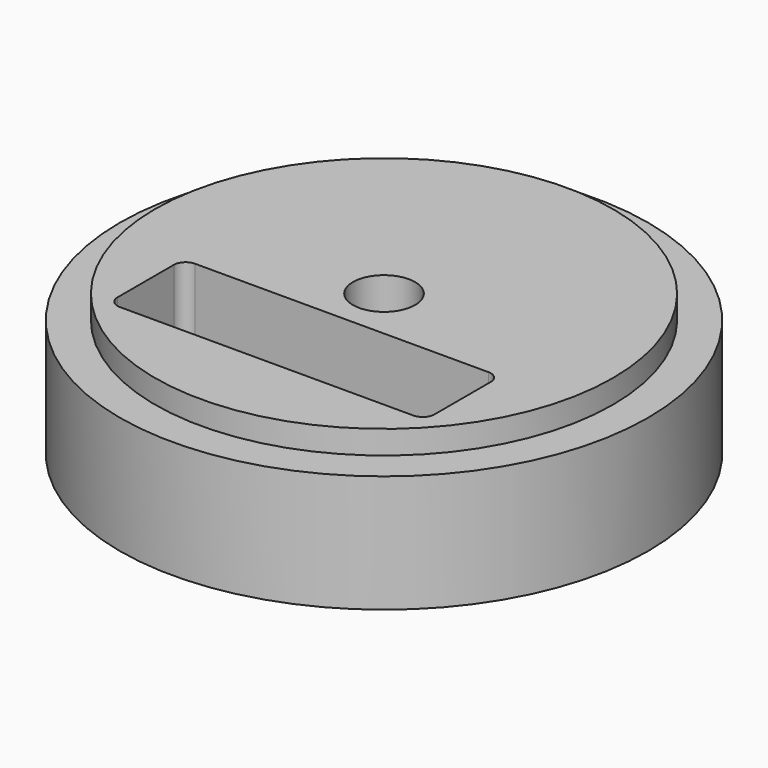
from build123d import *

# Parameters (mm, degrees)
F0_R     = 22.5
F1_DEPTH = 10
F3_R     = 19.5
F4_DEPTH = 2
F5_R     = 2.65
F5_W     = 27
F5_H     = 8
F6_DEPTH = 12.001
F8_R     = 1


with BuildPart() as f1:
    # F0 (on Top) → F1 (new body)
    with BuildSketch(Plane.XY):
        Circle(F0_R)
    extrude(amount=F1_DEPTH)

    # F3 (on face) → F4 (join)
    with BuildSketch(Plane.XY.offset(10)):
        Circle(F3_R)
    extrude(amount=F4_DEPTH)

    # F5 (on face) → F6 (cut, through all)
    with BuildSketch(Plane.XY.offset(12)):
        Circle(F5_R)
        with Locations((0, -8.5)):
            Rectangle(F5_W, F5_H)
    extrude(amount=-F6_DEPTH, mode=Mode.SUBTRACT)

    # F8
    f8_edges = [f1.edges().sort_by_distance(p)[0] for p in [
        (-13.5, -12.5, 6),
        (-13.5, -4.5, 6),
        (13.5, -4.5, 6),
        (13.5, -12.5, 6),
    ]]
    fillet(f8_edges, radius=F8_R)


solid = f1.part
